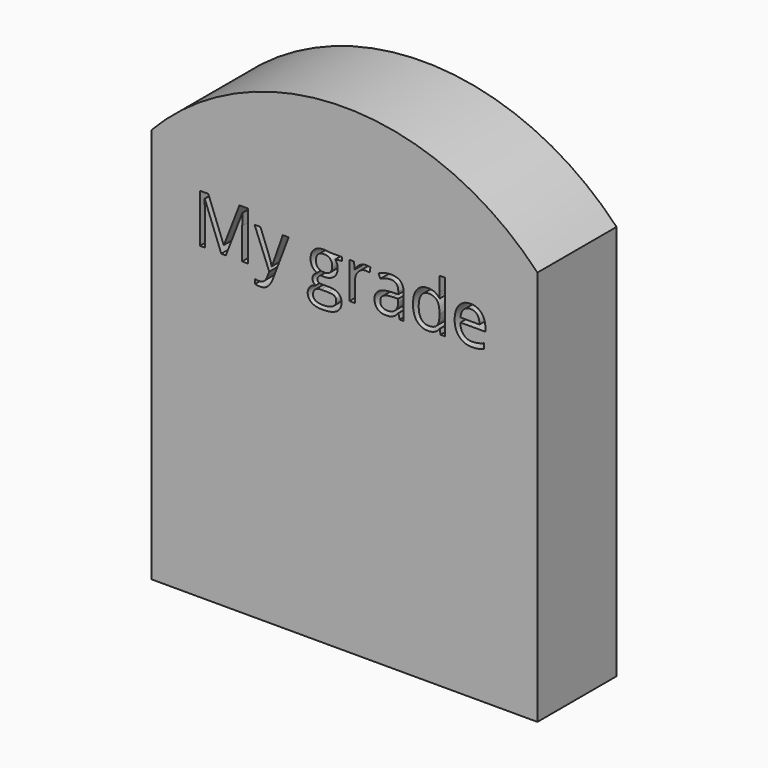
from build123d import *

# Parameters (mm, degrees)
F1_DEPTH     = 25.4
F2_TEXT_SIZE = 17.4564198017
F3_DEPTH     = 15.494


# Not quite as in the source:
# - Text() gives the source's letters only with a copy of the font that has no kerning and outlines rounded to 1/6400 em; it was checked with that copy


with BuildPart() as f1:
    # F0 (on Front) → F1 (new body)
    with BuildSketch(Plane.XZ):
        with BuildLine():
            Line((-44.8208354241, 54.4635542668), (-44.8208354241, -47.1364457332))
            Line((-44.8208354241, -47.1364457332), (54.3184257871, -47.1364457332))
            Line((54.3184257871, -47.1364457332), (54.3184257871, 54.4635542668))
            ThreePointArc((54.3184257871, 54.4635542668), (4.7487951815, 75.7440953473), (-44.8208354241, 54.4635542668))
        make_face()
    extrude(amount=F1_DEPTH)

    # F2 (on face) → F3 (cut)
    with BuildSketch(Plane.XZ.offset(25.4)):
        with Locations((-34.114831343, 32.3193142097)):
            Text('My grade', F2_TEXT_SIZE, font='Open Sans', text_align=(TextAlign.LEFT, TextAlign.BOTTOM))
    extrude(amount=-F3_DEPTH, mode=Mode.SUBTRACT)


solid = f1.part
